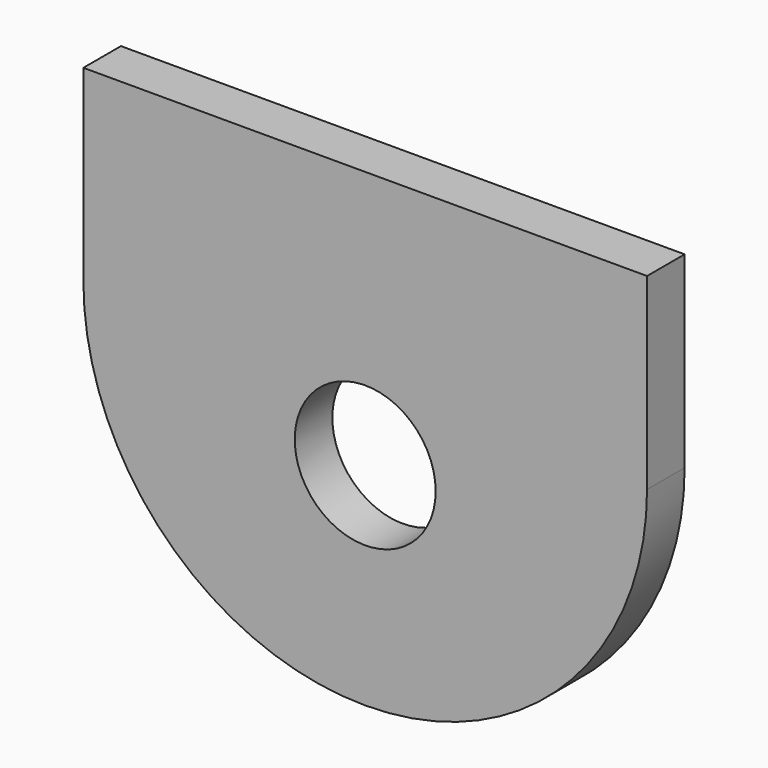
from build123d import *

# Parameters (mm, degrees)
F0_W     = 120
F0_H     = 100
F1_DEPTH = 10
F2_R     = 15
F3_DEPTH = 10.001
F4_R     = 59.99999


# Not quite as in the source:
# - a fillet or chamfer is up to 0.001 mm smaller than in the source, because OpenCascade refuses the exact size


with BuildPart() as f1:
    # F0 (on Front) → F1 (new body)
    with BuildSketch(Plane.XZ):
        Rectangle(F0_W, F0_H)
    extrude(amount=-F1_DEPTH)

    # F2 (on Front) → F3 (cut, through all)
    with BuildSketch(Plane.XZ):
        with Locations((0, -5)):
            Circle(F2_R)
    extrude(amount=-F3_DEPTH, mode=Mode.SUBTRACT)

    # F4 (radius 60 in the source; OpenCascade refuses exactly that, so slightly less here)
    f4_edges = [f1.edges().sort_by_distance(p)[0] for p in [
        (-60, 5, -50),
        (60, 5, -50),
    ]]
    fillet(f4_edges, radius=F4_R)


solid = f1.part
